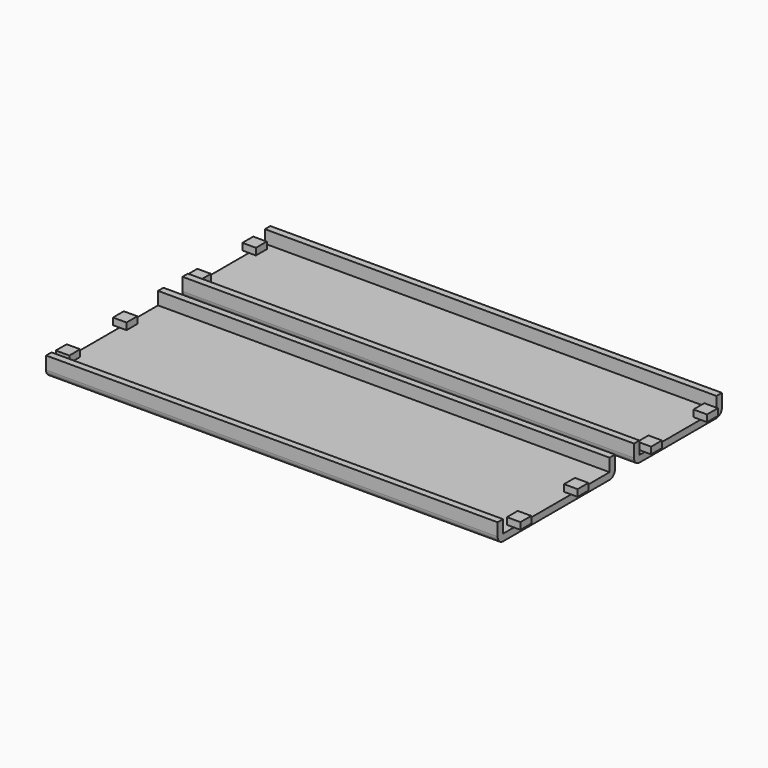
from build123d import *

# Parameters (mm, degrees)
F1_DEPTH = 84.6709
F2_START = 82.042
F0_W     = 5.08
F0_H     = 2.54
F2_DEPTH = 5.08
F3_START = -82.042
F3_DEPTH = 5.08


with BuildPart() as f1:
    # F0 (on Right) → F1 (new body, symmetric)
    with BuildSketch(Plane.YZ):
        with BuildLine():
            Line((18.2118, 169.3418), (15.6718, 169.3418))
            Line((15.6718, 169.3418), (15.6718, 164.5491375))
            ThreePointArc((15.6718, 164.5491375), (16.4157487758, 162.7530862758), (18.2118, 162.0091375))
            Line((18.2118, 162.0091375), (68.1474244764, 162.0091375))
            ThreePointArc((68.1474244764, 162.0091375), (68.3044763435, 162.0139975214), (68.4609272063, 162.0285589874))
            Line((68.4609272063, 162.0285589874), (69.6856973646, 162.9407926238))
            Line((69.6856973646, 162.9407926238), (68.1474244764, 165.0060867035))
            Line((68.1474244764, 165.0060867035), (68.1474244764, 164.5491375))
            Line((68.1474244764, 164.5491375), (55.1748093832, 164.5491375))
            Line((55.1748093832, 164.5491375), (50.0948093832, 164.5491375))
            Line((50.0948093832, 164.5491375), (28.3718, 164.5491375))
            Line((28.3718, 164.5491375), (23.2918, 164.5491375))
            Line((23.2918, 164.5491375), (18.2118, 164.5491375))
            Line((18.2118, 164.5491375), (18.2118, 169.3418))
        make_face()
        with BuildLine():
            Line((70.6874244764, 169.3418), (68.1474244764, 169.3418))
            Line((68.1474244764, 169.3418), (68.1474244764, 165.0060867035))
            Line((68.1474244764, 165.0060867035), (69.6856973646, 162.9407926238))
            Line((69.6856973646, 162.9407926238), (68.4609272063, 162.0285589874))
            ThreePointArc((68.4609272063, 162.0285589874), (70.0510915867, 162.8675752701), (70.6874244764, 164.5491375))
            Line((70.6874244764, 164.5491375), (70.6874244764, 165.8480664454))
            Line((70.6874244764, 165.8480664454), (70.6874244764, 169.3418))
        make_face()
    extrude(amount=F1_DEPTH, both=True)

    # F0 (on Right) → F2 (join)
    with BuildSketch(Plane.YZ.offset(F2_START)):
        with Locations((52.6348093832, 165.8191375)):
            Rectangle(F0_W, F0_H)
        Polygon((23.2918, 167.0891375), (23.2918, 164.5491375), (28.3718, 164.5491375), (28.3718, 167.0891375), align=None)
    extrude(amount=F2_DEPTH)

    # F0 (on Right) → F3 (join)
    with BuildSketch(Plane.YZ.offset(F3_START)):
        Polygon((23.2918, 167.0891375), (23.2918, 164.5491375), (28.3718, 164.5491375), (28.3718, 167.0891375), align=None)
        with Locations((52.6348093832, 165.8191375)):
            Rectangle(F0_W, F0_H)
    extrude(amount=-F3_DEPTH)


with BuildPart() as f1b:
    # F0 (on Right) → F1, piece 2 (new body, symmetric)
    with BuildSketch(Plane.YZ):
        with BuildLine():
            Line((82.1398573303, 169.3418), (79.5998573303, 169.3418))
            Line((79.5998573303, 169.3418), (79.5998573303, 164.5491375))
            ThreePointArc((79.5998573303, 164.5491375), (80.3438061061, 162.7530862758), (82.1398573303, 162.0091375))
            Line((82.1398573303, 162.0091375), (100.203, 162.0091375))
            Line((100.203, 162.0091375), (100.203, 164.5491375))
            Line((100.203, 164.5491375), (89.6502663064, 164.5491375))
            Line((89.6502663064, 164.5491375), (84.5702663064, 164.5491375))
            Line((84.5702663064, 164.5491375), (82.1398573303, 164.5491375))
            Line((82.1398573303, 164.5491375), (82.1398573303, 169.3418))
        make_face()
        with BuildLine():
            Line((120.8061426697, 169.3418), (118.2661426697, 169.3418))
            Line((118.2661426697, 169.3418), (118.2661426697, 164.5491375))
            Line((118.2661426697, 164.5491375), (115.8357336936, 164.5491375))
            Line((115.8357336936, 164.5491375), (110.7557336936, 164.5491375))
            Line((110.7557336936, 164.5491375), (100.203, 164.5491375))
            Line((100.203, 164.5491375), (100.203, 162.0091375))
            Line((100.203, 162.0091375), (118.2661426697, 162.0091375))
            ThreePointArc((118.2661426697, 162.0091375), (120.0621938939, 162.7530862758), (120.8061426697, 164.5491375))
            Line((120.8061426697, 164.5491375), (120.8061426697, 169.3418))
        make_face()
    extrude(amount=F1_DEPTH, both=True)

    # F0 (on Right) → F2, piece 2 (join)
    with BuildSketch(Plane.YZ.offset(F2_START)):
        with Locations((87.1102663064, 165.8191375)):
            Rectangle(F0_W, F0_H)
        with Locations((113.2957336936, 165.8191375)):
            Rectangle(F0_W, F0_H)
    extrude(amount=F2_DEPTH)

    # F0 (on Right) → F3, piece 2 (join)
    with BuildSketch(Plane.YZ.offset(F3_START)):
        with Locations((87.1102663064, 165.8191375)):
            Rectangle(F0_W, F0_H)
        with Locations((113.2957336936, 165.8191375)):
            Rectangle(F0_W, F0_H)
    extrude(amount=-F3_DEPTH)


solid = Compound([f1.part, f1b.part])
